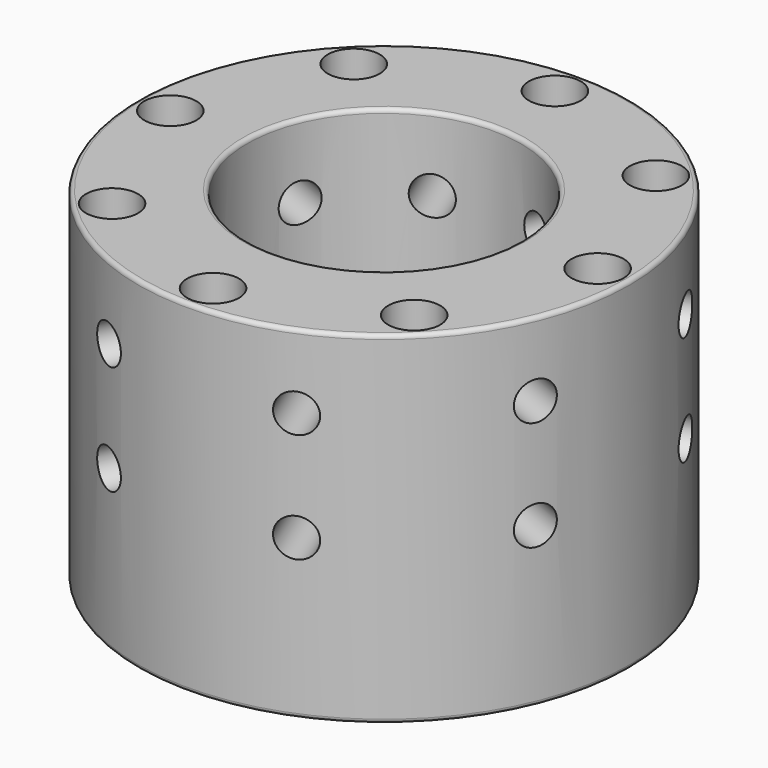
from build123d import *

# Parameters (mm, degrees)
F0_R             = 22.7965
F1_DEPTH         = 31.75
F2_R             = 15.24
F3_DEPTH         = 12.7
F4_R             = 12.7
F5_DEPTH         = 19.051
F6_R             = 0.381
F8_R             = 2.413
F9_DEPTH         = 31.751
F11_R            = 1.778
F12_DEPTH        = 38.1
F12_COPIES_COUNT = 4
F12_COPIES_ANGLE = 135


# Not quite as in the source:
# - a pattern or mirror of a feature is missing from the dataset's text; its kind, count and spacing are read off the source's solid


with BuildPart() as f1:
    # F0 (on Top) → F1 (new body)
    with BuildSketch(Plane.XY):
        Circle(F0_R)
    extrude(amount=F1_DEPTH)

    # F2 (on face) → F3 (cut)
    with BuildSketch(Plane(origin=(0, 0, 0), x_dir=(1, 0, 0), z_dir=(0, 0, -1))):
        Circle(F2_R)
    extrude(amount=-F3_DEPTH, mode=Mode.SUBTRACT)

    # F4 (on face) → F5 (cut, through all)
    with BuildSketch(Plane(origin=(0, 0, 12.7), x_dir=(1, 0, 0), z_dir=(0, 0, -1))):
        Circle(F4_R)
    extrude(amount=-F5_DEPTH, mode=Mode.SUBTRACT)

    # F6
    f6_edges = [f1.edges().sort_by_distance(p)[0] for p in [
        (-22.7965, 0, 31.75),
        (-12.7, 0, 31.75),
        (-22.7965, 0, 0),
        (-15.24, 0, 0),
        (-12.7, 0, 12.7),
        (-15.24, 0, 12.7),
    ]]
    fillet(f6_edges, radius=F6_R)

    # F8 (on face) → F9 (cut, through all)
    with BuildSketch(Plane(origin=(0, 0, 0), x_dir=(1, 0, 0), z_dir=(0, 0, -1))):
        with Locations((0, 19.812)):
            Circle(F8_R)
        with Locations((-14.0091995489, 14.0091995489)):
            Circle(F8_R)
        with Locations((-19.812, 0)):
            Circle(F8_R)
        with Locations((-14.0091995489, -14.0091995489)):
            Circle(F8_R)
        with Locations((0, -19.812)):
            Circle(F8_R)
        with Locations((14.0091995489, -14.0091995489)):
            Circle(F8_R)
        with Locations((19.812, 0)):
            Circle(F8_R)
        with Locations((14.0091995489, 14.0091995489)):
            Circle(F8_R)
    extrude(amount=-F9_DEPTH, mode=Mode.SUBTRACT)

    # F11 (on line) → F12 (cut, symmetric)
    with BuildSketch(Plane(origin=(0, 0, 0), x_dir=(-0.3826834324, 0.9238795325, 0), z_dir=(0.9238795325, 0.3826834324, 0))):
        with Locations((0, 24.892)):
            Circle(F11_R)
        with Locations((0, 14.732)):
            Circle(F11_R)
    f12 = extrude(amount=F12_DEPTH, both=True, mode=Mode.SUBTRACT)

    # F12_copies: F12 ×4 about axis
    f12_copies_axis = Axis((-2e-06, -1.4e-05, 0), (0, 0, -1))
    for i in range(1, F12_COPIES_COUNT):
        add(f12.rotate(f12_copies_axis, i * F12_COPIES_ANGLE / (F12_COPIES_COUNT - 1)), mode=Mode.SUBTRACT)


solid = f1.part
